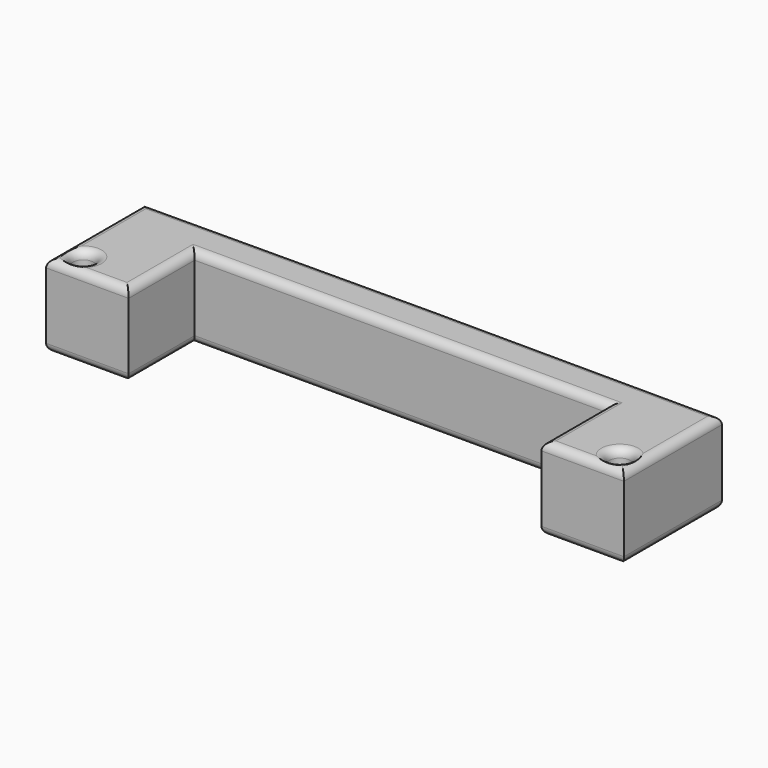
from build123d import *

# Parameters (mm, degrees)
F1_DEPTH     = 20
F3_D         = 5
F5_T1_DEPTH  = 39.6866504653
F5_T3_DEPTH  = 75.0024143135
F5_T5_DEPTH  = 75.0024143135
F5_T7_DEPTH  = 30.0041054994
F5_T9_DEPTH  = 25.0024143135
F5_T11_DEPTH = 100
F5_T13_DEPTH = 30.0041054994
F5_T27_DEPTH = 30.004828627
F5_T31_DEPTH = 105.0024143135
F5_T38_DEPTH = 105.0024143135
F5_T42_DEPTH = 30.004828627
F5_T49_DEPTH = 105.0024143135
F5_T53_DEPTH = 30.004828627
F5_T60_DEPTH = 30.004828627
F5_T64_DEPTH = 105.0024143135


# Not quite as in the source:
# - a fillet or chamfer that OpenCascade refuses, or shapes differently, is made with other operations: its cross-section is extruded or revolved along the edge and cut away or added


with BuildPart() as f1:
    # F0 (on Top) → F1 (new body)
    with BuildSketch(Plane.XY):
        Polygon((69.9992768724, 29.6818218383), (0, 30), (0, 20), (50, 20), (50, 0), (69.9992768724, 0), align=None)
    extrude(amount=F1_DEPTH)

    # F3 (through all)
    with Locations(Plane.XY.offset(20)):
        with Locations((64.9992768724, 5)):
            Hole(F3_D / 2)

    # F4: F1 across face


with BuildPart() as f1_1:
    add(f1.part)
    add(f1.part.mirror(Plane(origin=(0, 25, 10), x_dir=(0, -1, 0), z_dir=(-1, 0, 0))))

    # F5: fillet of radius 2 on 22 edges, made by hand

    # F5_s2 → F5_t1 (cut)
    with BuildSketch(Plane.XZ.offset(-34.6842361518)):
        with BuildLine():
            ThreePointArc((69.9996768724, 17.9990343146), (69.4134904348, 19.4142135624), (67.998311187, 20.0004))
            Line((67.998311187, 20.0004), (67.998311187, 20.2005365685))
            ThreePointArc((67.998311187, 20.2005365685), (68.9987940297, 20.2001365685), (69.9992768724, 20.2001365685))
            Line((69.9992768724, 20.2001365685), (70.1994134409, 20))
            ThreePointArc((70.1994134409, 20), (70.1994134409, 18.9995171573), (70.1998134409, 17.9990343146))
            Line((70.1998134409, 17.9990343146), (69.9996768724, 17.9990343146))
        make_face()
        with BuildLine():
            ThreePointArc((-67.998311187, 20.0004), (-69.4134904348, 19.4142135624), (-69.9996768724, 17.9990343146))
            Line((-69.9996768724, 17.9990343146), (-70.1998134409, 17.9990343146))
            ThreePointArc((-70.1998134409, 17.9990343146), (-70.1994134409, 18.9995171573), (-70.1994134409, 20))
            Line((-70.1994134409, 20), (-69.9992768724, 20.2001365685))
            ThreePointArc((-69.9992768724, 20.2001365685), (-68.9987940297, 20.2001365685), (-67.998311187, 20.2005365685))
            Line((-67.998311187, 20.2005365685), (-67.998311187, 20.0004))
        make_face()
        with BuildLine():
            ThreePointArc((69.9996768724, 2.0009656854), (69.4134904348, 0.5857864376), (67.998311187, -0.0004))
            Line((67.998311187, -0.0004), (67.998311187, -0.2005365685))
            ThreePointArc((67.998311187, -0.2005365685), (68.9987940297, -0.2001365685), (69.9992768724, -0.2001365685))
            Line((69.9992768724, -0.2001365685), (70.1994134409, 0))
            ThreePointArc((70.1994134409, 0), (70.1994134409, 1.0004828427), (70.1998134409, 2.0009656854))
            Line((70.1998134409, 2.0009656854), (69.9996768724, 2.0009656854))
        make_face()
        with BuildLine():
            ThreePointArc((-69.9996768724, 2.0009656854), (-69.4134904348, 0.5857864376), (-67.998311187, -0.0004))
            Line((-67.998311187, -0.0004), (-67.998311187, -0.2005365685))
            ThreePointArc((-67.998311187, -0.2005365685), (-68.9987940297, -0.2001365685), (-69.9992768724, -0.2001365685))
            Line((-69.9992768724, -0.2001365685), (-70.1994134409, 0))
            ThreePointArc((-70.1994134409, 0), (-70.1994134409, 1.0004828427), (-70.1998134409, 2.0009656854))
            Line((-70.1998134409, 2.0009656854), (-69.9996768724, 2.0009656854))
        make_face()
    extrude(amount=F5_T1_DEPTH, mode=Mode.SUBTRACT)

    # F5_s4 → F5_t3 (cut)
    with BuildSketch(Plane(origin=(74.8652788484, -0.3402963268, 0), x_dir=(0, 0, 1), z_dir=(-0.9999896696, 0.0045454023, 0))):
        with BuildLine():
            ThreePointArc((20.0004, 27.9987244027), (19.4142135624, 29.4139036505), (17.9990343146, 30.0000900882))
            Line((17.9990343146, 30.0000900882), (17.9990343146, 30.2002266567))
            ThreePointArc((17.9990343146, 30.2002266567), (18.9995171573, 30.1998266567), (20, 30.1998266567))
            Line((20, 30.1998266567), (20.2001365685, 29.9996900882))
            ThreePointArc((20.2001365685, 29.9996900882), (20.2001365685, 28.9992072455), (20.2005365685, 27.9987244027))
            Line((20.2005365685, 27.9987244027), (20.0004, 27.9987244027))
        make_face()
        with BuildLine():
            ThreePointArc((-0.0004, 27.9987244027), (0.5857864376, 29.4139036505), (2.0009656854, 30.0000900882))
            Line((2.0009656854, 30.0000900882), (2.0009656854, 30.2002266567))
            ThreePointArc((2.0009656854, 30.2002266567), (1.0004828427, 30.1998266567), (0, 30.1998266567))
            Line((0, 30.1998266567), (-0.2001365685, 29.9996900882))
            ThreePointArc((-0.2001365685, 29.9996900882), (-0.2001365685, 28.9992072455), (-0.2005365685, 27.9987244027))
            Line((-0.2005365685, 27.9987244027), (-0.0004, 27.9987244027))
        make_face()
    extrude(amount=F5_T3_DEPTH, mode=Mode.SUBTRACT)

    # F5_s6 → F5_t5 (cut)
    with BuildSketch(Plane(origin=(-74.8652788484, -0.3402963268, 0), x_dir=(0, 0, 1), z_dir=(0.9999896696, 0.0045454023, 0))):
        with BuildLine():
            ThreePointArc((20.0004, -27.9987244027), (19.4142135624, -29.4139036505), (17.9990343146, -30.0000900882))
            Line((17.9990343146, -30.0000900882), (17.9990343146, -30.2002266567))
            ThreePointArc((17.9990343146, -30.2002266567), (18.9995171573, -30.1998266567), (20, -30.1998266567))
            Line((20, -30.1998266567), (20.2001365685, -29.9996900882))
            ThreePointArc((20.2001365685, -29.9996900882), (20.2001365685, -28.9992072455), (20.2005365685, -27.9987244027))
            Line((20.2005365685, -27.9987244027), (20.0004, -27.9987244027))
        make_face()
        with BuildLine():
            ThreePointArc((2.0009656854, -30.0000900882), (0.5857864376, -29.4139036505), (-0.0004, -27.9987244027))
            Line((-0.0004, -27.9987244027), (-0.2005365685, -27.9987244027))
            ThreePointArc((-0.2005365685, -27.9987244027), (-0.2001365685, -28.9992072455), (-0.2001365685, -29.9996900882))
            Line((-0.2001365685, -29.9996900882), (0, -30.1998266567))
            ThreePointArc((0, -30.1998266567), (1.0004828427, -30.1998266567), (2.0009656854, -30.2002266567))
            Line((2.0009656854, -30.2002266567), (2.0009656854, -30.0000900882))
        make_face()
    extrude(amount=F5_T5_DEPTH, mode=Mode.SUBTRACT)

    # F5_s8 → F5_t7 (cut)
    with BuildSketch(Plane.YZ.offset(-75.0016911859)):
        with BuildLine():
            ThreePointArc((2.0009656854, 20.0004), (0.5857864376, 19.4142135624), (-0.0004, 17.9990343146))
            Line((-0.0004, 17.9990343146), (-0.2005365685, 17.9990343146))
            ThreePointArc((-0.2005365685, 17.9990343146), (-0.2001365685, 18.9995171573), (-0.2001365685, 20))
            Line((-0.2001365685, 20), (0, 20.2001365685))
            ThreePointArc((0, 20.2001365685), (1.0004828427, 20.2001365685), (2.0009656854, 20.2005365685))
            Line((2.0009656854, 20.2005365685), (2.0009656854, 20.0004))
        make_face()
        with BuildLine():
            ThreePointArc((-0.0004, 2.0009656854), (0.5857864376, 0.5857864376), (2.0009656854, -0.0004))
            Line((2.0009656854, -0.0004), (2.0009656854, -0.2005365685))
            ThreePointArc((2.0009656854, -0.2005365685), (1.0004828427, -0.2001365685), (0, -0.2001365685))
            Line((0, -0.2001365685), (-0.2001365685, 0))
            ThreePointArc((-0.2001365685, 0), (-0.2001365685, 1.0004828427), (-0.2005365685, 2.0009656854))
            Line((-0.2005365685, 2.0009656854), (-0.0004, 2.0009656854))
        make_face()
    extrude(amount=F5_T7_DEPTH, mode=Mode.SUBTRACT)

    # F5_s10 → F5_t9 (cut)
    with BuildSketch(Plane.XZ.offset(-20)):
        with BuildLine():
            ThreePointArc((-52.0009656854, 20.0004), (-50.5857864376, 19.4142135624), (-49.9996, 17.9990343146))
            Line((-49.9996, 17.9990343146), (-49.7994634315, 17.9990343146))
            ThreePointArc((-49.7994634315, 17.9990343146), (-49.7998634315, 18.9995171573), (-49.7998634315, 20))
            Line((-49.7998634315, 20), (-50, 20.2001365685))
            ThreePointArc((-50, 20.2001365685), (-51.0004828427, 20.2001365685), (-52.0009656854, 20.2005365685))
            Line((-52.0009656854, 20.2005365685), (-52.0009656854, 20.0004))
        make_face()
        with BuildLine():
            ThreePointArc((52.0009656854, 20.0004), (50.5857864376, 19.4142135624), (49.9996, 17.9990343146))
            Line((49.9996, 17.9990343146), (49.7994634315, 17.9990343146))
            ThreePointArc((49.7994634315, 17.9990343146), (49.7998634315, 18.9995171573), (49.7998634315, 20))
            Line((49.7998634315, 20), (50, 20.2001365685))
            ThreePointArc((50, 20.2001365685), (51.0004828427, 20.2001365685), (52.0009656854, 20.2005365685))
            Line((52.0009656854, 20.2005365685), (52.0009656854, 20.0004))
        make_face()
        with BuildLine():
            ThreePointArc((-49.9996, 2.0009656854), (-50.5857864376, 0.5857864376), (-52.0009656854, -0.0004))
            Line((-52.0009656854, -0.0004), (-52.0009656854, -0.2005365685))
            ThreePointArc((-52.0009656854, -0.2005365685), (-51.0004828427, -0.2001365685), (-50, -0.2001365685))
            Line((-50, -0.2001365685), (-49.7998634315, 0))
            ThreePointArc((-49.7998634315, 0), (-49.7998634315, 1.0004828427), (-49.7994634315, 2.0009656854))
            Line((-49.7994634315, 2.0009656854), (-49.9996, 2.0009656854))
        make_face()
        with BuildLine():
            ThreePointArc((49.9996, 2.0009656854), (50.5857864376, 0.5857864376), (52.0009656854, -0.0004))
            Line((52.0009656854, -0.0004), (52.0009656854, -0.2005365685))
            ThreePointArc((52.0009656854, -0.2005365685), (51.0004828427, -0.2001365685), (50, -0.2001365685))
            Line((50, -0.2001365685), (49.7998634315, 0))
            ThreePointArc((49.7998634315, 0), (49.7998634315, 1.0004828427), (49.7994634315, 2.0009656854))
            Line((49.7994634315, 2.0009656854), (49.9996, 2.0009656854))
        make_face()
    extrude(amount=F5_T9_DEPTH, mode=Mode.SUBTRACT)

    # F5_s12 → F5_t11 (cut)
    with BuildSketch(Plane.YZ.offset(-50)):
        with BuildLine():
            ThreePointArc((22.0009656854, 20.0004), (20.5857864376, 19.4142135624), (19.9996, 17.9990343146))
            Line((19.9996, 17.9990343146), (19.7994634315, 17.9990343146))
            ThreePointArc((19.7994634315, 17.9990343146), (19.7998634315, 18.9995171573), (19.7998634315, 20))
            Line((19.7998634315, 20), (20, 20.2001365685))
            ThreePointArc((20, 20.2001365685), (21.0004828427, 20.2001365685), (22.0009656854, 20.2005365685))
            Line((22.0009656854, 20.2005365685), (22.0009656854, 20.0004))
        make_face()
        with BuildLine():
            ThreePointArc((19.9996, 2.0009656854), (20.5857864376, 0.5857864376), (22.0009656854, -0.0004))
            Line((22.0009656854, -0.0004), (22.0009656854, -0.2005365685))
            ThreePointArc((22.0009656854, -0.2005365685), (21.0004828427, -0.2001365685), (20, -0.2001365685))
            Line((20, -0.2001365685), (19.7998634315, 0))
            ThreePointArc((19.7998634315, 0), (19.7998634315, 1.0004828427), (19.7994634315, 2.0009656854))
            Line((19.7994634315, 2.0009656854), (19.9996, 2.0009656854))
        make_face()
    extrude(amount=F5_T11_DEPTH, mode=Mode.SUBTRACT)

    # F5_s14 → F5_t13 (cut)
    with BuildSketch(Plane.YZ.offset(44.9975856865)):
        with BuildLine():
            ThreePointArc((2.0009656854, 20.0004), (0.5857864376, 19.4142135624), (-0.0004, 17.9990343146))
            Line((-0.0004, 17.9990343146), (-0.2005365685, 17.9990343146))
            ThreePointArc((-0.2005365685, 17.9990343146), (-0.2001365685, 18.9995171573), (-0.2001365685, 20))
            Line((-0.2001365685, 20), (0, 20.2001365685))
            ThreePointArc((0, 20.2001365685), (1.0004828427, 20.2001365685), (2.0009656854, 20.2005365685))
            Line((2.0009656854, 20.2005365685), (2.0009656854, 20.0004))
        make_face()
        with BuildLine():
            ThreePointArc((2.0009656854, -0.0004), (0.5857864376, 0.5857864376), (-0.0004, 2.0009656854))
            Line((-0.0004, 2.0009656854), (-0.2005365685, 2.0009656854))
            ThreePointArc((-0.2005365685, 2.0009656854), (-0.2001365685, 1.0004828427), (-0.2001365685, 0))
            Line((-0.2001365685, 0), (0, -0.2001365685))
            ThreePointArc((0, -0.2001365685), (1.0004828427, -0.2001365685), (2.0009656854, -0.2005365685))
            Line((2.0009656854, -0.2005365685), (2.0009656854, -0.0004))
        make_face()
    extrude(amount=F5_T13_DEPTH, mode=Mode.SUBTRACT)

    # F5_s15 → F5_t16 (revolve, cut)
    with BuildSketch(Plane.XZ.offset(-5)):
        with BuildLine():
            ThreePointArc((69.5002425578, 20.0004), (68.08506331, 19.4142135624), (67.4988768724, 17.9990343146))
            Line((67.4988768724, 17.9990343146), (67.2987403038, 17.9990343146))
            ThreePointArc((67.2987403038, 17.9990343146), (67.2991403038, 18.9995171573), (67.2991403038, 20))
            Line((67.2991403038, 20), (67.4992768724, 20.2001365685))
            ThreePointArc((67.4992768724, 20.2001365685), (68.4997597151, 20.2001365685), (69.5002425578, 20.2005365685))
            Line((69.5002425578, 20.2005365685), (69.5002425578, 20.0004))
        make_face()
    revolve(axis=Axis((64.9992768724, 5, 20), (0, 0, 1)), mode=Mode.SUBTRACT)

    # F5_s17 → F5_t18 (revolve, cut)
    with BuildSketch(Plane.XZ.offset(-5)):
        with BuildLine():
            ThreePointArc((-69.5002425578, 20.0004), (-68.08506331, 19.4142135624), (-67.4988768724, 17.9990343146))
            Line((-67.4988768724, 17.9990343146), (-67.2987403038, 17.9990343146))
            ThreePointArc((-67.2987403038, 17.9990343146), (-67.2991403038, 18.9995171573), (-67.2991403038, 20))
            Line((-67.2991403038, 20), (-67.4992768724, 20.2001365685))
            ThreePointArc((-67.4992768724, 20.2001365685), (-68.4997597151, 20.2001365685), (-69.5002425578, 20.2005365685))
            Line((-69.5002425578, 20.2005365685), (-69.5002425578, 20.0004))
        make_face()
    revolve(axis=Axis((-64.9992768724, 5, 20), (0, 0, -1)), mode=Mode.SUBTRACT)

    # F5_s19 → F5_t20 (revolve, cut)
    with BuildSketch(Plane.XZ.offset(-5)):
        with BuildLine():
            ThreePointArc((67.4988768724, 2.0009656854), (68.08506331, 0.5857864376), (69.5002425578, -0.0004))
            Line((69.5002425578, -0.0004), (69.5002425578, -0.2005365685))
            ThreePointArc((69.5002425578, -0.2005365685), (68.4997597151, -0.2001365685), (67.4992768724, -0.2001365685))
            Line((67.4992768724, -0.2001365685), (67.2991403038, 0))
            ThreePointArc((67.2991403038, 0), (67.2991403038, 1.0004828427), (67.2987403038, 2.0009656854))
            Line((67.2987403038, 2.0009656854), (67.4988768724, 2.0009656854))
        make_face()
    revolve(axis=Axis((64.9992768724, 5, 0), (0, 0, 1)), mode=Mode.SUBTRACT)

    # F5_s21 → F5_t22 (revolve, cut)
    with BuildSketch(Plane.XZ.offset(-5)):
        with BuildLine():
            ThreePointArc((-67.4988768724, 2.0009656854), (-68.08506331, 0.5857864376), (-69.5002425578, -0.0004))
            Line((-69.5002425578, -0.0004), (-69.5002425578, -0.2005365685))
            ThreePointArc((-69.5002425578, -0.2005365685), (-68.4997597151, -0.2001365685), (-67.4992768724, -0.2001365685))
            Line((-67.4992768724, -0.2001365685), (-67.2991403038, 0))
            ThreePointArc((-67.2991403038, 0), (-67.2991403038, 1.0004828427), (-67.2987403038, 2.0009656854))
            Line((-67.2987403038, 2.0009656854), (-67.4988768724, 2.0009656854))
        make_face()
    revolve(axis=Axis((-64.9992768724, 5, 0), (0, 0, -1)), mode=Mode.SUBTRACT)


with BuildPart() as f5_tool25:
    # F5_s26 → F5_t27 (new body)
    with BuildSketch(Plane.XZ.offset(-25.0024143135)):
        with BuildLine():
            ThreePointArc((-52.0009656854, 20.0004), (-50.5857864376, 19.4142135624), (-49.9996, 17.9990343146))
            Line((-49.9996, 17.9990343146), (-49.7994634315, 17.9990343146))
            ThreePointArc((-49.7994634315, 17.9990343146), (-49.7998634315, 18.9995171573), (-49.7998634315, 20))
            Line((-49.7998634315, 20), (-50, 20.2001365685))
            ThreePointArc((-50, 20.2001365685), (-51.0004828427, 20.2001365685), (-52.0009656854, 20.2005365685))
            Line((-52.0009656854, 20.2005365685), (-52.0009656854, 20.0004))
        make_face()
    extrude(amount=F5_T27_DEPTH)

    split(bisect_by=Plane.XZ.offset(-20), keep=Keep.BOTTOM)


with BuildPart() as f5_tool29:
    # F5_s30 → F5_t31 (new body)
    with BuildSketch(Plane.YZ.offset(-55.0024143135)):
        with BuildLine():
            ThreePointArc((22.0009656854, 20.0004), (20.5857864376, 19.4142135624), (19.9996, 17.9990343146))
            Line((19.9996, 17.9990343146), (19.7994634315, 17.9990343146))
            ThreePointArc((19.7994634315, 17.9990343146), (19.7998634315, 18.9995171573), (19.7998634315, 20))
            Line((19.7998634315, 20), (20, 20.2001365685))
            ThreePointArc((20, 20.2001365685), (21.0004828427, 20.2001365685), (22.0009656854, 20.2005365685))
            Line((22.0009656854, 20.2005365685), (22.0009656854, 20.0004))
        make_face()
    extrude(amount=F5_T31_DEPTH)

    split(bisect_by=Plane.YZ.offset(-50), keep=Keep.BOTTOM)


with BuildPart() as f5_tool25_1:
    add(f5_tool25.part)

    # F5_t33: intersect F5_tool29
    add(f5_tool29.part, mode=Mode.INTERSECT)


with BuildPart() as f1_2:
    add(f1_1.part)

    # F5_t23: cut F5_tool25
    add(f5_tool25_1.part, mode=Mode.SUBTRACT)


with BuildPart() as f5_tool36:
    # F5_s37 → F5_t38 (new body)
    with BuildSketch(Plane.YZ.offset(-50)):
        with BuildLine():
            ThreePointArc((22.0009656854, 20.0004), (20.5857864376, 19.4142135624), (19.9996, 17.9990343146))
            Line((19.9996, 17.9990343146), (19.7994634315, 17.9990343146))
            ThreePointArc((19.7994634315, 17.9990343146), (19.7998634315, 18.9995171573), (19.7998634315, 20))
            Line((19.7998634315, 20), (20, 20.2001365685))
            ThreePointArc((20, 20.2001365685), (21.0004828427, 20.2001365685), (22.0009656854, 20.2005365685))
            Line((22.0009656854, 20.2005365685), (22.0009656854, 20.0004))
        make_face()
    extrude(amount=F5_T38_DEPTH)

    split(bisect_by=Plane.YZ.offset(50), keep=Keep.TOP)


with BuildPart() as f5_tool40:
    # F5_s41 → F5_t42 (new body)
    with BuildSketch(Plane.XZ.offset(-25.0024143135)):
        with BuildLine():
            ThreePointArc((52.0009656854, 20.0004), (50.5857864376, 19.4142135624), (49.9996, 17.9990343146))
            Line((49.9996, 17.9990343146), (49.7994634315, 17.9990343146))
            ThreePointArc((49.7994634315, 17.9990343146), (49.7998634315, 18.9995171573), (49.7998634315, 20))
            Line((49.7998634315, 20), (50, 20.2001365685))
            ThreePointArc((50, 20.2001365685), (51.0004828427, 20.2001365685), (52.0009656854, 20.2005365685))
            Line((52.0009656854, 20.2005365685), (52.0009656854, 20.0004))
        make_face()
    extrude(amount=F5_T42_DEPTH)

    split(bisect_by=Plane.XZ.offset(-20), keep=Keep.BOTTOM)


with BuildPart() as f5_tool36_1:
    add(f5_tool36.part)

    # F5_t44: intersect F5_tool40
    add(f5_tool40.part, mode=Mode.INTERSECT)


with BuildPart() as f1_3:
    add(f1_2.part)

    # F5_t34: cut F5_tool36
    add(f5_tool36_1.part, mode=Mode.SUBTRACT)


with BuildPart() as f5_tool47:
    # F5_s48 → F5_t49 (new body)
    with BuildSketch(Plane.YZ.offset(50)):
        with BuildLine():
            ThreePointArc((19.9996, 2.0009656854), (20.5857864376, 0.5857864376), (22.0009656854, -0.0004))
            Line((22.0009656854, -0.0004), (22.0009656854, -0.2005365685))
            ThreePointArc((22.0009656854, -0.2005365685), (21.0004828427, -0.2001365685), (20, -0.2001365685))
            Line((20, -0.2001365685), (19.7998634315, 0))
            ThreePointArc((19.7998634315, 0), (19.7998634315, 1.0004828427), (19.7994634315, 2.0009656854))
            Line((19.7994634315, 2.0009656854), (19.9996, 2.0009656854))
        make_face()
    extrude(amount=-F5_T49_DEPTH)

    split(bisect_by=Plane.YZ.offset(-50), keep=Keep.BOTTOM)


with BuildPart() as f5_tool51:
    # F5_s52 → F5_t53 (new body)
    with BuildSketch(Plane.XZ.offset(-25.0024143135)):
        with BuildLine():
            ThreePointArc((-49.9996, 2.0009656854), (-50.5857864376, 0.5857864376), (-52.0009656854, -0.0004))
            Line((-52.0009656854, -0.0004), (-52.0009656854, -0.2005365685))
            ThreePointArc((-52.0009656854, -0.2005365685), (-51.0004828427, -0.2001365685), (-50, -0.2001365685))
            Line((-50, -0.2001365685), (-49.7998634315, 0))
            ThreePointArc((-49.7998634315, 0), (-49.7998634315, 1.0004828427), (-49.7994634315, 2.0009656854))
            Line((-49.7994634315, 2.0009656854), (-49.9996, 2.0009656854))
        make_face()
    extrude(amount=F5_T53_DEPTH)

    split(bisect_by=Plane.XZ.offset(-20), keep=Keep.BOTTOM)


with BuildPart() as f5_tool47_1:
    add(f5_tool47.part)

    # F5_t55: intersect F5_tool51
    add(f5_tool51.part, mode=Mode.INTERSECT)


with BuildPart() as f1_4:
    add(f1_3.part)

    # F5_t45: cut F5_tool47
    add(f5_tool47_1.part, mode=Mode.SUBTRACT)


with BuildPart() as f5_tool58:
    # F5_s59 → F5_t60 (new body)
    with BuildSketch(Plane.XZ.offset(-25.0024143135)):
        with BuildLine():
            ThreePointArc((49.9996, 2.0009656854), (50.5857864376, 0.5857864376), (52.0009656854, -0.0004))
            Line((52.0009656854, -0.0004), (52.0009656854, -0.2005365685))
            ThreePointArc((52.0009656854, -0.2005365685), (51.0004828427, -0.2001365685), (50, -0.2001365685))
            Line((50, -0.2001365685), (49.7998634315, 0))
            ThreePointArc((49.7998634315, 0), (49.7998634315, 1.0004828427), (49.7994634315, 2.0009656854))
            Line((49.7994634315, 2.0009656854), (49.9996, 2.0009656854))
        make_face()
    extrude(amount=F5_T60_DEPTH)

    split(bisect_by=Plane.XZ.offset(-20), keep=Keep.BOTTOM)


with BuildPart() as f5_tool62:
    # F5_s63 → F5_t64 (new body)
    with BuildSketch(Plane.YZ.offset(55.0024143135)):
        with BuildLine():
            ThreePointArc((19.9996, 2.0009656854), (20.5857864376, 0.5857864376), (22.0009656854, -0.0004))
            Line((22.0009656854, -0.0004), (22.0009656854, -0.2005365685))
            ThreePointArc((22.0009656854, -0.2005365685), (21.0004828427, -0.2001365685), (20, -0.2001365685))
            Line((20, -0.2001365685), (19.7998634315, 0))
            ThreePointArc((19.7998634315, 0), (19.7998634315, 1.0004828427), (19.7994634315, 2.0009656854))
            Line((19.7994634315, 2.0009656854), (19.9996, 2.0009656854))
        make_face()
    extrude(amount=-F5_T64_DEPTH)

    split(bisect_by=Plane.YZ.offset(50), keep=Keep.TOP)


with BuildPart() as f5_tool58_1:
    add(f5_tool58.part)

    # F5_t66: intersect F5_tool62
    add(f5_tool62.part, mode=Mode.INTERSECT)


with BuildPart() as f1_5:
    add(f1_4.part)

    # F5_t56: cut F5_tool58
    add(f5_tool58_1.part, mode=Mode.SUBTRACT)


solid = f1_5.part
